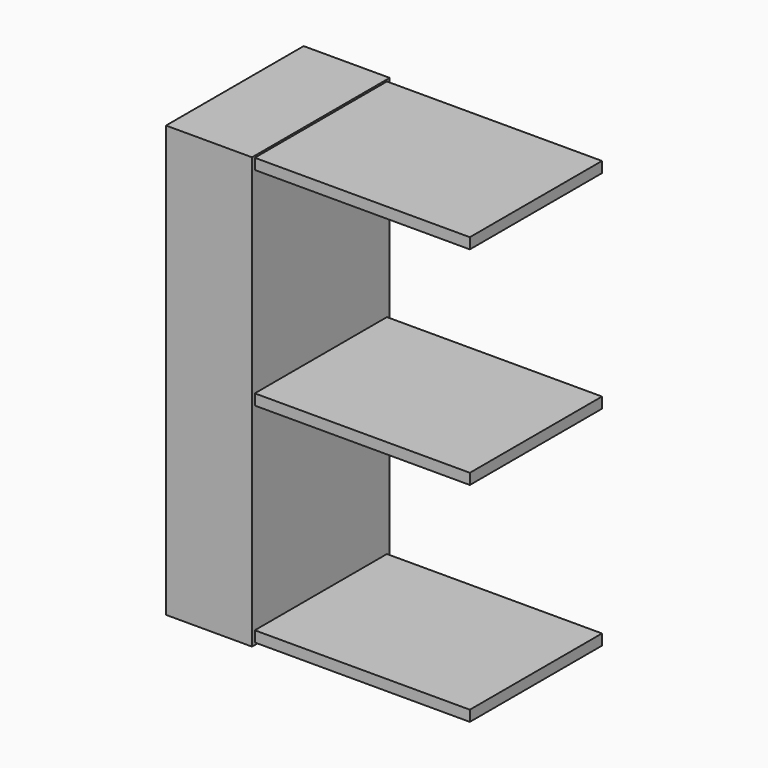
from build123d import *

# Parameters (mm, degrees)
F1_DEPTH      = 152.4
F1_DEPTH_BACK = 152.4
F2_W          = 381.0055409819
F2_H          = 19.05
F2_W_2        = 381
F3_DEPTH      = 6.096
F4_W          = 381.0055409819
F4_H          = 19.05
F4_W_2        = 381
F5_DEPTH      = 6.096


# Not quite as in the source:
# - ends of sketch curves that miss each other by under 0.0002 mm in the source are joined


with BuildPart() as f1:
    # F0 (on Front) → F1 (new body, two sides)
    with BuildSketch(Plane.XZ) as f1_sk:
        Polygon((-533.4, -382.5126007106), (-381, -382.5126007106), (-381, -378.4719215088), (0, -378.4719215088), (0, -359.4219215088), (-381, -359.4219215088), (-381, -356.2469204928), (-381, -12.157774965), (-381, -8.982775981), (0.0055409819, -8.982775981), (0.0055409819, 10.067224019), (-381, 10.067224019), (-381, 13.242225035), (-381, 355.2765448173), (-381, 358.4515458333), (0.0055409819, 358.4515458333), (0.0055409819, 377.5015458333), (-381, 377.5015458333), (-381, 380.6765448173), (-533.4, 380.6765468493), align=None)
    extrude(amount=F1_DEPTH)
    extrude(f1_sk.sketch, amount=-F1_DEPTH_BACK)

    # F2 (on face) → F3 (cut)
    with BuildSketch(Plane(origin=(0, 152.4, 0), x_dir=(-1, 0, 0), z_dir=(0, 1, 0))):
        with Locations((190.4972295091, 367.9765458333)):
            Rectangle(F2_W, F2_H)
        with Locations((190.4972295091, 0.542224019)):
            Rectangle(F2_W, F2_H)
        with Locations((190.5, -368.9469215088)):
            Rectangle(F2_W_2, F2_H)
    extrude(amount=-F3_DEPTH, mode=Mode.SUBTRACT)

    # F4 (on face) → F5 (cut)
    with BuildSketch(Plane.XZ.offset(152.4)):
        with Locations((-190.4972295091, 0.542224019)):
            Rectangle(F4_W, F4_H)
        with Locations((-190.4972295091, 367.9765458333)):
            Rectangle(F4_W, F4_H)
        with Locations((-190.5, -368.9469215088)):
            Rectangle(F4_W_2, F4_H)
    extrude(amount=-F5_DEPTH, mode=Mode.SUBTRACT)


solid = f1.part
